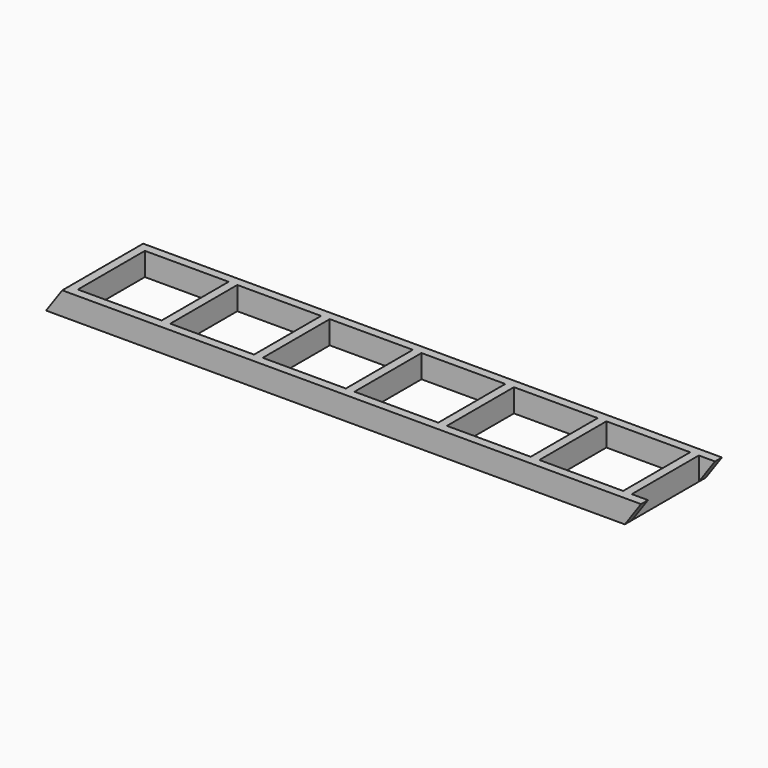
from build123d import *

# Parameters (mm, degrees)
F1_DEPTH = 38.1
F2_W     = 38.1
F2_H     = 101.6
F3_DEPTH = 368.3
F4_W     = 38.1
F4_H     = 101.6
F5_DEPTH = 38.1


# Not quite as in the source:
# - a feature names something its author has since deleted; it is built from what else it names


with BuildPart() as f1:
    # F0 (on Front) → F1 (new body)
    with BuildSketch(Plane.XZ):
        Polygon((71.1410858821, 101.6), (0, 0), (2544.7625, 0), (2615.9035858821, 101.6), align=None)
    extrude(amount=F1_DEPTH)

    # F2 (on face) → F3 (join)
    with BuildSketch(Plane.XZ.offset(38.1)):
        with Locations((90.1910858821, 50.8)):
            Rectangle(F2_W, F2_H)
        with Locations((496.5910858821, 50.8)):
            Rectangle(F2_W, F2_H)
        with Locations((902.9910858821, 50.8)):
            Rectangle(F2_W, F2_H)
        with Locations((1306.5125, 50.8)):
            Rectangle(F2_W, F2_H)
        with Locations((1712.9125, 50.8)):
            Rectangle(F2_W, F2_H)
        with Locations((2119.3125, 50.8)):
            Rectangle(F2_W, F2_H)
        with Locations((2525.7125, 50.8)):
            Rectangle(F2_W, F2_H)
    extrude(amount=F3_DEPTH)

    # F4 (on face) → F5 (join)
    with BuildSketch(Plane.XZ.offset(406.4)):
        Polygon((2615.9035858821, 101.6), (109.2410858821, 101.6), (109.2410858821, 0), (2544.7625, 0), align=None)
        with Locations((90.1910858821, 50.8)):
            Rectangle(F4_W, F4_H)
        Polygon((71.1410858821, 101.6), (0, 0), (71.1410858821, 0), align=None)
    extrude(amount=F5_DEPTH)


solid = f1.part
